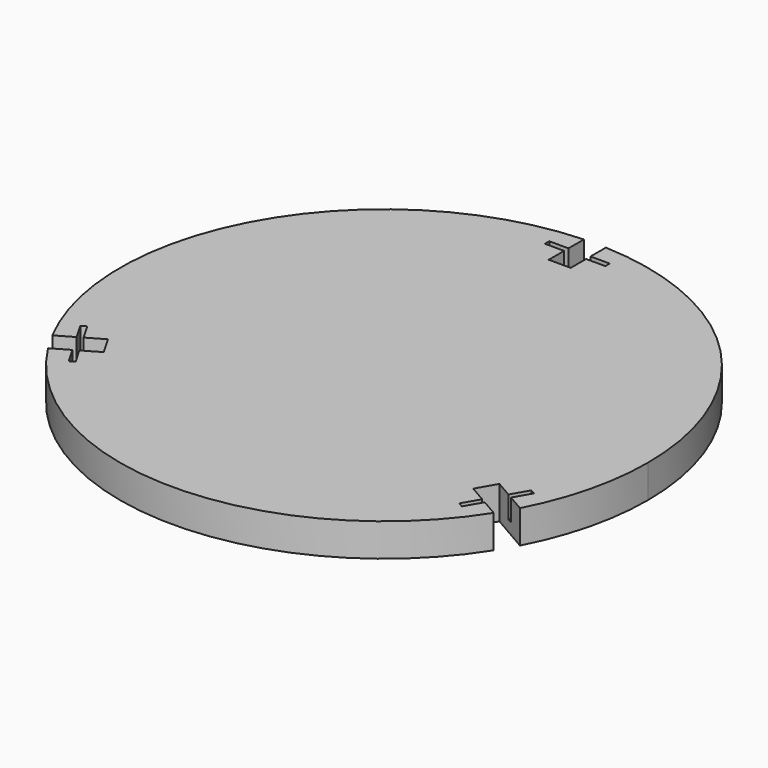
from build123d import *

# Parameters (mm, degrees)
F1_DEPTH        = 19.05
F2_W            = 3.175
F2_H            = 12.7
F3_DEPTH        = 17.4625
F3_COPIES_COUNT = 3


# Not quite as in the source:
# - a pattern or mirror of a feature is missing from the dataset's text; its kind, count and spacing are read off the source's solid


with BuildPart() as f1:
    # F0 (on Top) → F1 (new body)
    with BuildSketch(Plane.XY):
        with BuildLine():
            ThreePointArc((135.0426538238, -70.6345641186), (147.9970615295, -36.3679773788), (152.4, 0))
            ThreePointArc((152.4, 0), (109.9852262806, 105.4941230591), (6.35, 152.2676508652))
            Line((6.35, 152.2676508652), (6.35, 126.8676508652))
            Line((6.35, 126.8676508652), (-6.35, 126.8676508652))
            Line((-6.35, 126.8676508652), (-6.35, 152.2676508652))
            ThreePointArc((-6.35, 152.2676508652), (-131.9822715367, 76.2), (-135.0426538238, -70.6345641186))
            Line((-135.0426538238, -70.6345641186), (-113.0456085677, -57.9345641186))
            Line((-113.0456085677, -57.9345641186), (-106.6956085677, -68.9330867466))
            Line((-106.6956085677, -68.9330867466), (-128.6926538238, -81.6330867466))
            ThreePointArc((-128.6926538238, -81.6330867466), (0, -152.4), (128.6926538238, -81.6330867466))
            Line((128.6926538238, -81.6330867466), (106.6956085677, -68.9330867466))
            Line((106.6956085677, -68.9330867466), (113.0456085677, -57.9345641186))
            Line((113.0456085677, -57.9345641186), (135.0426538238, -70.6345641186))
        make_face()
    extrude(amount=F1_DEPTH)

    # F2 (on Right) → F3 (cut, symmetric)
    with BuildSketch(Plane.YZ):
        with Locations((139.5676508652, 12.7)):
            Rectangle(F2_W, F2_H)
    f3 = extrude(amount=F3_DEPTH, both=True, mode=Mode.SUBTRACT)

    # F3_copies: F3 ×3 about axis
    f3_copies_axis = Axis((0, 0, 0), (0, 0, 1))
    for i in range(1, F3_COPIES_COUNT):
        add(f3.rotate(f3_copies_axis, i * 360 / F3_COPIES_COUNT), mode=Mode.SUBTRACT)


solid = f1.part
